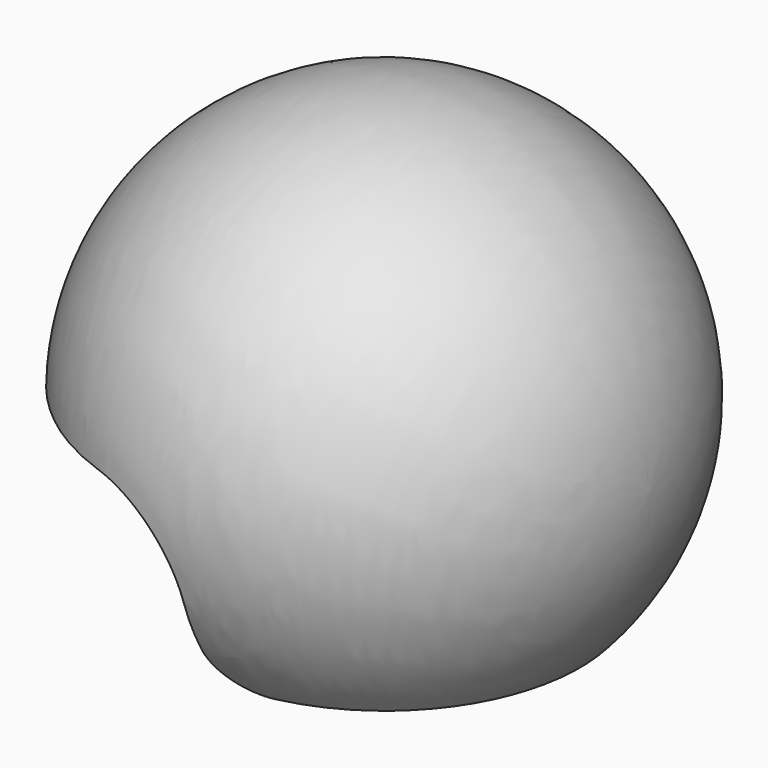
from build123d import *

# Parameters (mm, degrees)
F2_W        = 31.1245527118
F2_H        = 16.214504838
F3_DEPTH    = 68.58
F4_T1_DEPTH = 32.0391658923
F4_T3_DEPTH = 32.0391658923
F5_R        = 10.16


# Not quite as in the source:
# - a fillet or chamfer that OpenCascade refuses, or shapes differently, is made with other operations: its cross-section is extruded or revolved along the edge and cut away or added


with BuildPart() as f1:
    # F0 (on Front) → F1 (revolve)
    with BuildSketch(Plane.XZ):
        with BuildLine():
            Line((26.0988561893, 0.1960262089), (30.6322429805, 0.1960262089))
            ThreePointArc((30.6322429805, 0.1960262089), (0, 30.6328701935), (-30.6322429805, 0.1960262089))
            Line((-30.6322429805, 0.1960262089), (-26.0988561893, 0.1960262089))
            ThreePointArc((-26.0988561893, 0.1960262089), (0, 26.0995923467), (26.0988561893, 0.1960262089))
        make_face()
    revolve(axis=Axis((28.3655495849, 0, 0.1960262089), (-1, 0, 0)))

    # F2 (on Front) → F3 (cut, symmetric)
    with BuildSketch(Plane.XZ):
        Polygon((0, -20.2416591346), (0, 0.970325782), (-34.5226228237, 0.970325782), (-34.5226228237, -36.4561639726), (0, -36.4561639726), align=None)
        with Locations((15.5622763559, -28.3489115536)):
            Rectangle(F2_W, F2_H)
    extrude(amount=F3_DEPTH, both=True, mode=Mode.SUBTRACT)

    # F4: fillet of radius 5.08 on 2 edges, made by hand

    # F4_s2 → F4_t1 (cut)
    with BuildSketch(Plane.XZ.offset(-35.254433922)):
        with BuildLine():
            ThreePointArc((0, -15.1616591346), (1.4878975516, -18.7537615831), (5.08, -20.2416591346))
            Line((5.08, -20.2416591346), (0, -20.2416591346))
            Line((0, -20.2416591346), (0, -15.1616591346))
        make_face()
    extrude(amount=F4_T1_DEPTH, mode=Mode.SUBTRACT)

    # F4_s4 → F4_t3 (cut)
    with BuildSketch(Plane.XZ.offset(3.2152680297)):
        with BuildLine():
            ThreePointArc((5.08, -20.2416591346), (1.4878975516, -18.7537615831), (0, -15.1616591346))
            Line((0, -15.1616591346), (0, -20.2416591346))
            Line((0, -20.2416591346), (5.08, -20.2416591346))
        make_face()
    extrude(amount=F4_T3_DEPTH, mode=Mode.SUBTRACT)

    # F5
    f5_edges = [f1.edges().sort_by_distance(p)[0] for p in [
        (0, 28.159492, 0.970326),
        (0, -28.159492, 0.970326),
    ]]
    fillet(f5_edges, radius=F5_R)


solid = f1.part
